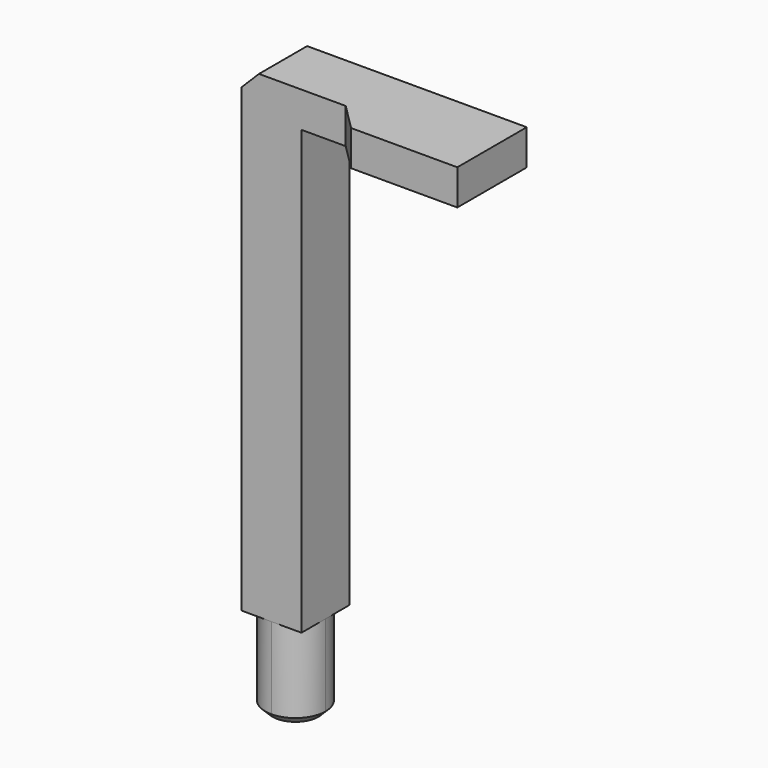
from build123d import *

# Parameters (mm, degrees)
F0_W        = 3.4
F0_H        = 3.4
F1_DEPTH    = 27
F2_SIZE     = 1
F3_W        = 4.9
F3_H        = 2
F4_DEPTH    = 10
F5_T4_DEPTH = 22.5734639037
F7_DEPTH    = 5


# Not quite as in the source:
# - a fillet or chamfer that OpenCascade refuses, or shapes differently, is made with other operations: its cross-section is extruded or revolved along the edge and cut away or added


with BuildPart() as f1:
    # F0 (on Top) → F1 (new body)
    with BuildSketch(Plane.XY):
        Rectangle(F0_W, F0_H)
    extrude(amount=F1_DEPTH)

    # F2
    f2_edges = [f1.edges().sort_by_distance(p)[0] for p in [
        (-1.7, 0, 27),
    ]]
    chamfer(f2_edges, length=F2_SIZE)

    # F3 (on face) → F4 (join)
    with BuildSketch(Plane.YZ.offset(1.7)):
        with Locations((-0.75, 26)):
            Rectangle(F3_W, F3_H)
    extrude(amount=F4_DEPTH)

    # F5: chamfer of 4 on 1 edges, made by hand


with BuildPart() as f5_tool2:
    # F5_s3 → F5_t4 (new body)
    with BuildSketch(Plane.XY.offset(37.2867319519)):
        Polygon((1.7, 0.8), (5.7, -3.2), (1.7, -3.2), align=None)
    extrude(amount=-F5_T4_DEPTH)

    split(bisect_by=Plane.XZ.offset(1.7), keep=Keep.TOP)


with BuildPart() as f1_1:
    add(f1.part)

    # F5_t1: cut F5_tool2
    add(f5_tool2.part, mode=Mode.SUBTRACT)

    # F6 (on face) → F7 (join)
    with BuildSketch(Plane.XY):
        with BuildLine():
            ThreePointArc((0, -1.7), (1.202081528, -1.202081528), (1.7, 0))
            ThreePointArc((1.7, 0), (1.202081528, 1.202081528), (0, 1.7))
            ThreePointArc((0, 1.7), (-1.202081528, 1.202081528), (-1.7, 0))
            ThreePointArc((-1.7, 0), (-1.202081528, -1.202081528), (0, -1.7))
        make_face()
    extrude(amount=-F7_DEPTH)

    # F8: chamfer of 0.4 on 1 edges, made by hand

    # F8_s1 → F8_t2 (revolve, cut)
    with BuildSketch(Plane.XZ):
        Polygon((-1.7, -4.6), (-1.3, -5), (-1.7, -5), align=None)
    revolve(axis=Axis((0, 0, -5), (0, 0, 1)), mode=Mode.SUBTRACT)


solid = f1_1.part
